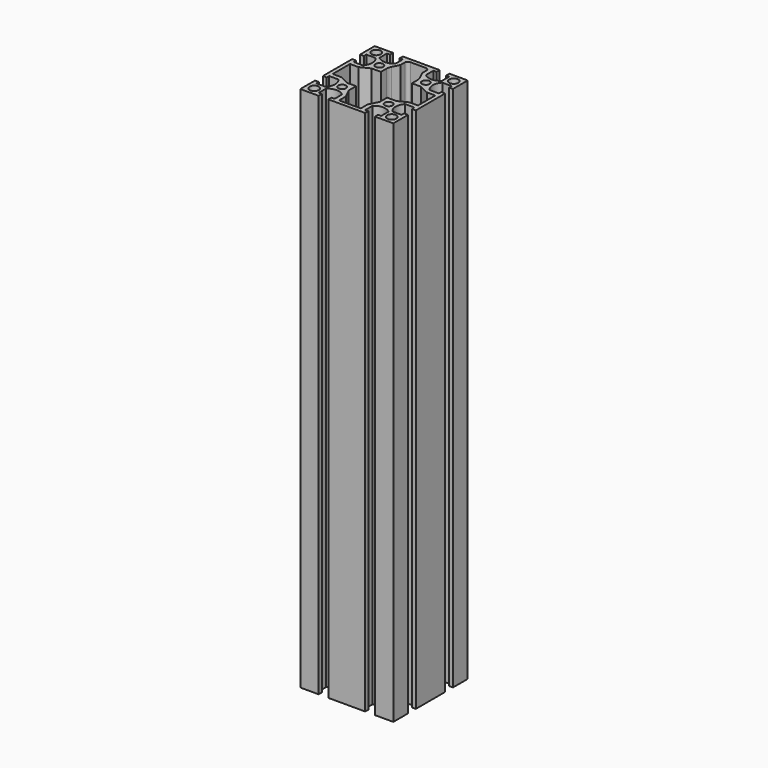
from build123d import *

# Parameters (mm, degrees)
F0_R     = 3
F0_R_2   = 2.5
F1_DEPTH = 340
F2_R     = 2
F3_R     = 7


# Not quite as in the source:
# - a feature names something its author has since deleted; it is built from what else it names


with BuildPart() as f1:
    # F0 (on Top) → F1 (new body)
    with BuildSketch(Plane.XY):
        with BuildLine():
            Line((18.15, -30), (30, -30))
            Line((30, -30), (30, -18.15))
            Line((30, -18.15), (27.5, -18.15))
            Line((27.5, -18.15), (27.5, -20.15))
            Line((27.5, -20.15), (21.5477069044, -20.15))
            ThreePointArc((21.5477069044, -20.15), (19.5, -15), (21.5477069044, -9.85))
            Line((21.5477069044, -9.85), (27.5, -9.85))
            Line((27.5, -9.85), (27.5, -11.85))
            Line((27.5, -11.85), (30, -11.85))
            Line((30, -11.85), (30, 11.85))
            Line((30, 11.85), (27.5, 11.85))
            Line((27.5, 11.85), (27.5, 9.85))
            Line((27.5, 9.85), (21.5477069044, 9.85))
            ThreePointArc((21.5477069044, 9.85), (19.5, 15), (21.5477069044, 20.15))
            Line((21.5477069044, 20.15), (27.5, 20.15))
            Line((27.5, 20.15), (27.5, 18.15))
            Line((27.5, 18.15), (30, 18.15))
            Line((30, 18.15), (30, 30))
            Line((30, 30), (18.15, 30))
            Line((18.15, 30), (18.15, 27.5))
            Line((18.15, 27.5), (20.15, 27.5))
            Line((20.15, 27.5), (20.15, 21.5477069044))
            ThreePointArc((20.15, 21.5477069044), (15, 19.5), (9.85, 21.5477069044))
            Line((9.85, 21.5477069044), (9.85, 27.5))
            Line((9.85, 27.5), (11.85, 27.5))
            Line((11.85, 27.5), (11.85, 30))
            Line((11.85, 30), (-11.85, 30))
            Line((-11.85, 30), (-11.85, 27.5))
            Line((-11.85, 27.5), (-9.85, 27.5))
            Line((-9.85, 27.5), (-9.85, 21.5477069044))
            ThreePointArc((-9.85, 21.5477069044), (-15, 19.5), (-20.15, 21.5477069044))
            Line((-20.15, 21.5477069044), (-20.15, 27.5))
            Line((-20.15, 27.5), (-18.15, 27.5))
            Line((-18.15, 27.5), (-18.15, 30))
            Line((-18.15, 30), (-30, 30))
            Line((-30, 30), (-30, 18.15))
            Line((-30, 18.15), (-27.5, 18.15))
            Line((-27.5, 18.15), (-27.5, 20.15))
            Line((-27.5, 20.15), (-21.5477069044, 20.15))
            ThreePointArc((-21.5477069044, 20.15), (-19.5, 15), (-21.5477069044, 9.85))
            Line((-21.5477069044, 9.85), (-27.5, 9.85))
            Line((-27.5, 9.85), (-27.5, 11.85))
            Line((-27.5, 11.85), (-30, 11.85))
            Line((-30, 11.85), (-30, -11.85))
            Line((-30, -11.85), (-27.5, -11.85))
            Line((-27.5, -11.85), (-27.5, -9.85))
            Line((-27.5, -9.85), (-21.5477069044, -9.85))
            ThreePointArc((-21.5477069044, -9.85), (-19.5, -15), (-21.5477069044, -20.15))
            Line((-21.5477069044, -20.15), (-27.5, -20.15))
            Line((-27.5, -20.15), (-27.5, -18.15))
            Line((-27.5, -18.15), (-30, -18.15))
            Line((-30, -18.15), (-30, -30))
            Line((-30, -30), (-18.15, -30))
            Line((-18.15, -30), (-18.15, -27.5))
            Line((-18.15, -27.5), (-20.15, -27.5))
            Line((-20.15, -27.5), (-20.15, -21.5477069044))
            ThreePointArc((-20.15, -21.5477069044), (-15, -19.5), (-9.85, -21.5477069044))
            Line((-9.85, -21.5477069044), (-9.85, -27.5))
            Line((-9.85, -27.5), (-11.85, -27.5))
            Line((-11.85, -27.5), (-11.85, -30))
            Line((-11.85, -30), (11.85, -30))
            Line((11.85, -30), (11.85, -27.5))
            Line((11.85, -27.5), (9.85, -27.5))
            Line((9.85, -27.5), (9.85, -21.5477069044))
            ThreePointArc((9.85, -21.5477069044), (15, -19.5), (20.15, -21.5477069044))
            Line((20.15, -21.5477069044), (20.15, -27.5))
            Line((20.15, -27.5), (18.15, -27.5))
            Line((18.15, -27.5), (18.15, -30))
        make_face()
        with Locations((-25, -25)):
            Circle(F0_R, mode=Mode.SUBTRACT)
        with Locations((-15, -15)):
            Circle(F0_R_2, mode=Mode.SUBTRACT)
        with Locations((25, -25)):
            Circle(F0_R, mode=Mode.SUBTRACT)
        with Locations((15, -15)):
            Circle(F0_R_2, mode=Mode.SUBTRACT)
        with Locations((-25, 25)):
            Circle(F0_R, mode=Mode.SUBTRACT)
        with Locations((-15, 15)):
            Circle(F0_R_2, mode=Mode.SUBTRACT)
        Polygon((-7, 22), (-7, 27.5), (0, 27.5), (7, 27.5), (7, 22), (10, 16), (10, 10), (16, 10), (22, 7), (27.5, 7), (27.5, 0), (27.5, -7), (22, -7), (16, -10), (10, -10), (10, -16), (7, -22), (7, -27.5), (0, -27.5), (-7, -27.5), (-7, -22), (-10, -16), (-10, -10), (-16, -10), (-22, -7), (-27.5, -7), (-27.5, 0), (-27.5, 7), (-22, 7), (-16, 10), (-10, 10), (-10, 16), align=None, mode=Mode.SUBTRACT)
        with Locations((15, 15)):
            Circle(F0_R_2, mode=Mode.SUBTRACT)
        with Locations((25, 25)):
            Circle(F0_R, mode=Mode.SUBTRACT)
    extrude(amount=F1_DEPTH)

    # F2
    f2_edges = [f1.edges().sort_by_distance(p)[0] for p in [
        (-7, 27.5, 170),
        (7, 27.5, 170),
    ]]
    fillet(f2_edges, radius=F2_R)

    # F3
    f3_edges = [f1.edges().sort_by_distance(p)[0] for p in [
        (-10, 16, 170),
        (10, 16, 170),
    ]]
    fillet(f3_edges, radius=F3_R)


solid = f1.part
